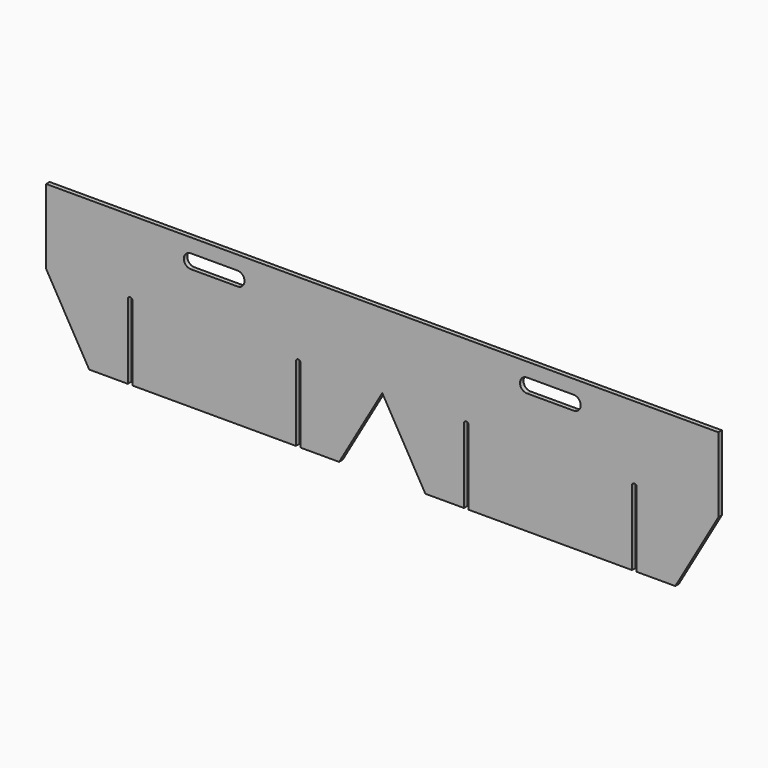
from build123d import *

# Parameters (mm, degrees)
F2_DEPTH = 11.90625


# Not quite as in the source:
# - a variable given as a bare number and used for a length is read in inches; the dataset says mm whatever the document's units were


with BuildPart() as f2:
    # F1 (on Front) → F2 (new body)
    with BuildSketch(Plane.XZ):
        with BuildLine():
            Line((914.4, 406.4), (0, 406.4))
            Line((0, 406.4), (0, 203.2))
            Line((0, 203.2), (117.3175746993, 0))
            Line((117.3175746993, 0), (222.25, 0))
            Line((222.25, 0), (222.25, 203.2))
            ThreePointArc((222.25, 203.2), (228.6, 209.55), (234.95, 203.2))
            Line((234.95, 203.2), (234.95, 0))
            Line((234.95, 0), (679.45, 0))
            Line((679.45, 0), (679.45, 203.2))
            ThreePointArc((679.45, 203.2), (685.8, 209.55), (692.15, 203.2))
            Line((692.15, 203.2), (692.15, 0))
            Line((692.15, 0), (797.0824253007, 0))
            Line((797.0824253007, 0), (914.4, 203.2))
            Line((914.4, 203.2), (1031.7175746993, 0))
            Line((1031.7175746993, 0), (1136.65, 0))
            Line((1136.65, 0), (1136.65, 203.2))
            ThreePointArc((1136.65, 203.2), (1143, 209.55), (1149.35, 203.2))
            Line((1149.35, 203.2), (1149.35, 0))
            Line((1149.35, 0), (1593.85, 0))
            Line((1593.85, 0), (1593.85, 203.2))
            ThreePointArc((1593.85, 203.2), (1600.2, 209.55), (1606.55, 203.2))
            Line((1606.55, 203.2), (1606.55, 0))
            Line((1606.55, 0), (1711.4824253007, 0))
            Line((1711.4824253007, 0), (1828.8, 203.2))
            Line((1828.8, 203.2), (1828.8, 406.4))
            Line((1828.8, 406.4), (914.4, 406.4))
        make_face()
        with BuildLine():
            Line((393.7, 368.3), (457.2, 368.3))
            Line((457.2, 368.3), (520.7, 368.3))
            ThreePointArc((520.7, 368.3), (539.75, 349.25), (520.7, 330.2))
            Line((520.7, 330.2), (457.2, 330.2))
            Line((457.2, 330.2), (393.7, 330.2))
            ThreePointArc((393.7, 330.2), (374.65, 349.25), (393.7, 368.3))
        make_face(mode=Mode.SUBTRACT)
        with BuildLine():
            Line((1308.1, 368.3), (1371.6, 368.3))
            Line((1371.6, 368.3), (1435.1, 368.3))
            ThreePointArc((1435.1, 368.3), (1454.15, 349.25), (1435.1, 330.2))
            Line((1435.1, 330.2), (1371.6, 330.2))
            Line((1371.6, 330.2), (1308.1, 330.2))
            ThreePointArc((1308.1, 330.2), (1289.05, 349.25), (1308.1, 368.3))
        make_face(mode=Mode.SUBTRACT)
    extrude(amount=F2_DEPTH)


solid = f2.part
